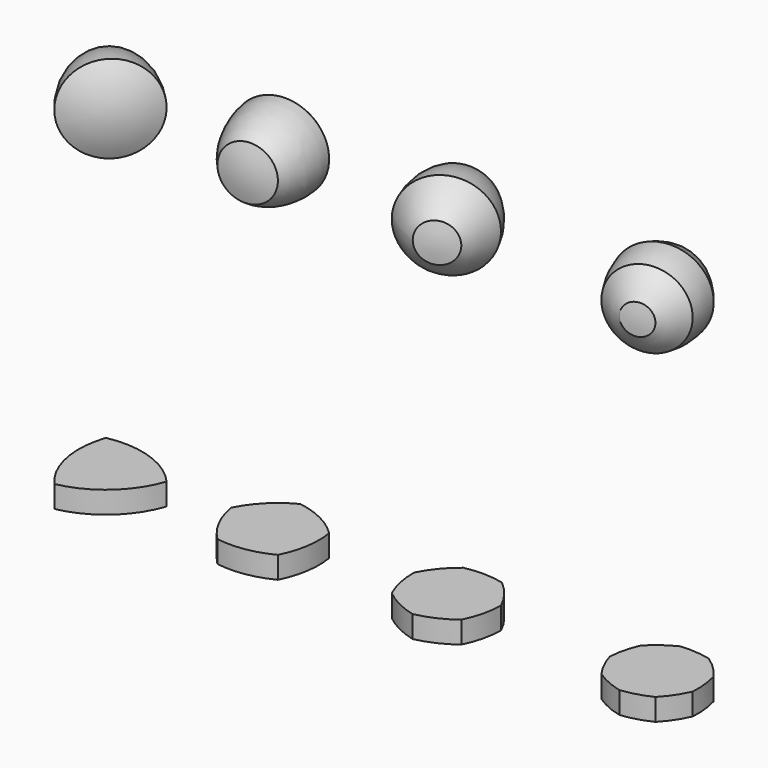
from build123d import *

# Parameters (mm, degrees)
F2_DEPTH = 6.35


# Not quite as in the source:
# - a variable given as a bare number and used for a length is read in inches; the dataset says mm whatever the document's units were


with BuildPart() as f2:
    # F1 (on Top) → F2 (new body)
    with BuildSketch(Plane.XY):
        with BuildLine():
            ThreePointArc((14.3781795579, 2.8846639207), (3.433975334, 10.1712608559), (-9.6872820156, 11.0095367969))
            ThreePointArc((-9.6872820156, 11.0095367969), (-10.5255579567, -2.1117205527), (-4.6908975422, -13.8942007176))
            ThreePointArc((-4.6908975422, -13.8942007176), (7.0915826227, -8.0595403031), (14.3781795579, 2.8846639207))
        make_face()
    extrude(amount=F2_DEPTH)


with BuildPart() as f2b:
    # F1 (on Top) → F2, piece 2 (new body)
    with BuildSketch(Plane.XY):
        with BuildLine():
            ThreePointArc((44.8035849855, 13.1835004697), (38.3870157524, 8.4951750576), (33.7332679985, 2.0534836852))
            ThreePointArc((33.7332679985, 2.0534836852), (36.2093014936, -5.4978085238), (40.8976269057, -11.9143777569))
            ThreePointArc((40.8976269057, -11.9143777569), (48.8444689961, -11.8930075889), (56.3957612051, -9.4169740938))
            ThreePointArc((56.3957612051, -9.4169740938), (58.8311462251, -1.8524743946), (58.8097760571, 6.0943676958))
            ThreePointArc((58.8097760571, 6.0943676958), (52.3680846847, 10.7481154497), (44.8035849855, 13.1835004697))
        make_face()
    extrude(amount=F2_DEPTH)


with BuildPart() as f2c:
    # F1 (on Top) → F2, piece 3 (new body)
    with BuildSketch(Plane.XY):
        with BuildLine():
            ThreePointArc((104.3052545657, 11.6467493191), (98.6638719794, 12.371883009), (93.0025732068, 11.8235103614))
            ThreePointArc((93.0025732068, 11.8235103614), (88.9182963481, 7.8650133115), (85.817269298, 3.096926946))
            ThreePointArc((85.817269298, 3.096926946), (86.3656419456, -2.5643718266), (88.1600232362, -7.9617056256))
            ThreePointArc((88.1600232362, -7.9617056256), (92.9281096017, -11.0627326756), (98.2666935225, -13.0250114719))
            ThreePointArc((98.2666935225, -13.0250114719), (103.6640273214, -11.2306301812), (108.5267512927, -8.2802180181))
            ThreePointArc((108.5267512927, -8.2802180181), (110.489030089, -2.9416340973), (111.2141637789, 2.699748489))
            ThreePointArc((111.2141637789, 2.699748489), (108.2637516157, 7.5624724603), (104.3052545657, 11.6467493191))
        make_face()
    extrude(amount=F2_DEPTH)


with BuildPart() as f2d:
    # F1 (on Top) → F2, piece 4 (new body)
    with BuildSketch(Plane.XY):
        with BuildLine():
            ThreePointArc((164.0093399435, 11.788726154), (159.6353220402, 12.4748948753), (155.2086033491, 12.3910989139))
            ThreePointArc((155.2086033491, 12.3910989139), (151.4168504878, 10.1051701371), (148.079650239, 7.1955387803))
            ThreePointArc((148.079650239, 7.1955387803), (146.6443657243, 3.0071239853), (145.958197003, -1.3668939181))
            ThreePointArc((145.958197003, -1.3668939181), (147.5509664107, -5.4979888997), (149.8368951876, -9.2897417609))
            ThreePointArc((149.8368951876, -9.2897417609), (153.7124440102, -11.4305316752), (157.9008588052, -12.8658161898))
            ThreePointArc((157.9008588052, -12.8658161898), (162.2457746766, -12.0146016436), (166.3768696582, -10.4218322359))
            ThreePointArc((166.3768696582, -10.4218322359), (169.1581181539, -6.9769059756), (171.2989080681, -3.101357153))
            ThreePointArc((171.2989080681, -3.101357153), (171.2151121068, 1.3253615381), (170.3638975606, 5.6702774095))
            ThreePointArc((170.3638975606, 5.6702774095), (167.4542662038, 9.0074776583), (164.0093399435, 11.788726154))
        make_face()
    extrude(amount=F2_DEPTH)


with BuildPart() as f5:
    # F4 (on offset) → F5 (revolve)
    with BuildSketch(Plane.XY.offset(101.6)):
        with BuildLine():
            Line((7.0915826227, -8.0595403031), (-9.6872820156, 11.0095367969))
            ThreePointArc((-9.6872820156, 11.0095367969), (-10.5255579567, -2.1117205527), (-4.6908975422, -13.8942007176))
            ThreePointArc((-4.6908975422, -13.8942007176), (1.5844163483, -11.7524669811), (7.0915826227, -8.0595403031))
        make_face()
    revolve(axis=Axis((-1.2978496965, 1.4749982469, 101.6), (0.660585222, -0.7507510669, 0)))


with BuildPart() as f6:
    # F4 (on offset) → F6 (revolve)
    with BuildSketch(Plane.XY.offset(101.6)):
        with BuildLine():
            ThreePointArc((44.8035849855, 13.1835004697), (38.3870157524, 8.4951750576), (33.7332679985, 2.0534836852))
            ThreePointArc((33.7332679985, 2.0534836852), (36.2093014936, -5.4978085238), (40.8976269057, -11.9143777569))
            ThreePointArc((40.8976269057, -11.9143777569), (44.8718888853, -12.2164076911), (48.8444689961, -11.8930075889))
            Line((48.8444689961, -11.8930075889), (44.8035849855, 13.1835004697))
        make_face()
    revolve(axis=Axis((46.8240269908, 0.6452464404, 101.6), (0.1590899217, -0.9872640968, 0)))


with BuildPart() as f7:
    # F4 (on offset) → F7 (revolve)
    with BuildSketch(Plane.XY.offset(101.6)):
        with BuildLine():
            Line((103.6640273214, -11.2306301812), (93.0025732068, 11.8235103614))
            ThreePointArc((93.0025732068, 11.8235103614), (88.9182963481, 7.8650133115), (85.817269298, 3.096926946))
            ThreePointArc((85.817269298, 3.096926946), (86.3656419456, -2.5643718266), (88.1600232362, -7.9617056256))
            ThreePointArc((88.1600232362, -7.9617056256), (92.9281096017, -11.0627326756), (98.2666935225, -13.0250114719))
            ThreePointArc((98.2666935225, -13.0250114719), (101.0157455678, -12.2793747089), (103.6640273214, -11.2306301812))
        make_face()
    revolve(axis=Axis((98.3333002641, 0.2964400901, 101.6), (0.419742288, -0.9076433285, 0)))


with BuildPart() as f8:
    # F4 (on offset) → F8 (revolve)
    with BuildSketch(Plane.XY.offset(101.6)):
        with BuildLine():
            Line((162.2457746766, -12.0146016436), (155.2086033491, 12.3910989139))
            ThreePointArc((155.2086033491, 12.3910989139), (151.4168504878, 10.1051701371), (148.079650239, 7.1955387803))
            ThreePointArc((148.079650239, 7.1955387803), (146.6443657243, 3.0071239853), (145.958197003, -1.3668939181))
            ThreePointArc((145.958197003, -1.3668939181), (147.5509664107, -5.4979888997), (149.8368951876, -9.2897417609))
            ThreePointArc((149.8368951876, -9.2897417609), (153.7124440102, -11.4305316752), (157.9008588052, -12.8658161898))
            ThreePointArc((157.9008588052, -12.8658161898), (160.0918991558, -12.5350604786), (162.2457746766, -12.0146016436))
        make_face()
    revolve(axis=Axis((158.7271890128, 0.1882486352, 101.6), (0.2770539893, -0.9608543527, 0)))


solid = Compound([f2.part, f2b.part, f2c.part, f2d.part, f5.part, f6.part, f7.part, f8.part])
